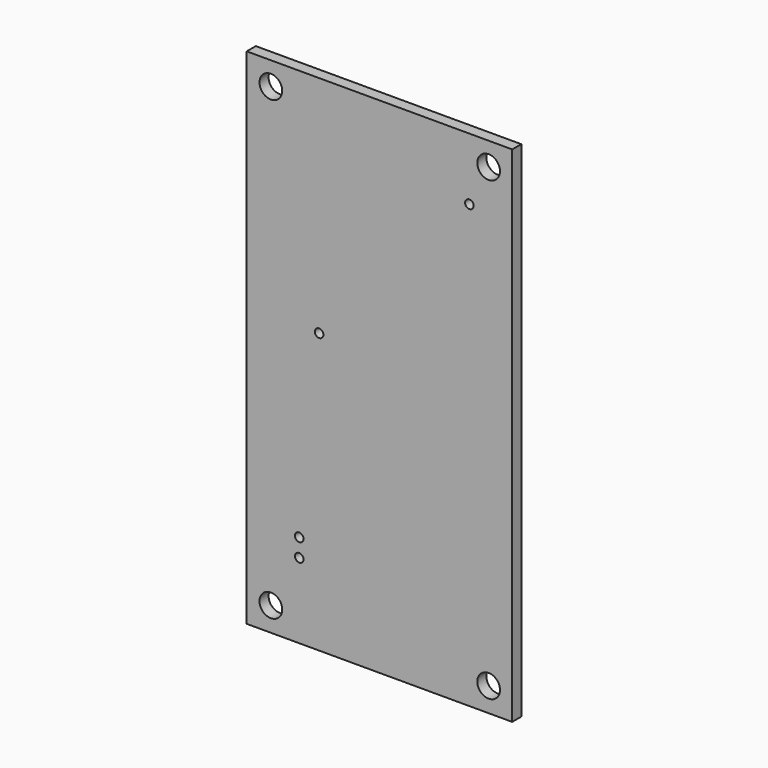
from build123d import *

# Parameters (mm, degrees)
F0_W         = 37.4
F0_H         = 71
F0_R         = 1.6
F0_R_2       = 0.6
F1_DEPTH     = 1.6
F2_TEXT_SIZE = 3.1366892573
F3_DEPTH     = 0.2


# Not quite as in the source:
# - Text() gives the source's letters only with a copy of the font that has no kerning and outlines rounded to 1/6400 em; it was checked with that copy


with BuildPart() as f1:
    # F0 (on Front) → F1 (new body)
    with BuildSketch(Plane.XZ):
        with Locations((18.7, 35.5)):
            Rectangle(F0_W, F0_H)
        with Locations((3.4, 3.4)):
            Circle(F0_R, mode=Mode.SUBTRACT)
        with Locations((7.4, 10.6)):
            Circle(F0_R_2, mode=Mode.SUBTRACT)
        with Locations((7.4, 13.14)):
            Circle(F0_R_2, mode=Mode.SUBTRACT)
        with Locations((34.08, 3.4)):
            Circle(F0_R, mode=Mode.SUBTRACT)
        with Locations((10.2, 39.36)):
            Circle(F0_R_2, mode=Mode.SUBTRACT)
        with Locations((3.4, 67.73)):
            Circle(F0_R, mode=Mode.SUBTRACT)
        with Locations((31.37, 62.24)):
            Circle(F0_R_2, mode=Mode.SUBTRACT)
        with Locations((34.08, 67.73)):
            Circle(F0_R, mode=Mode.SUBTRACT)
    extrude(amount=F1_DEPTH)

    # F2 (on face) → F3 (join)
    with BuildSketch(Plane(origin=(0, 0, 0), x_dir=(-1, 0, 0), z_dir=(0, 1, 0))):
        with Locations((-31.4918532968, 54.3432980776)):
            Text('<-NC', F2_TEXT_SIZE, font='Open Sans', text_align=(TextAlign.LEFT, TextAlign.BOTTOM))
    extrude(amount=F3_DEPTH)


solid = f1.part
